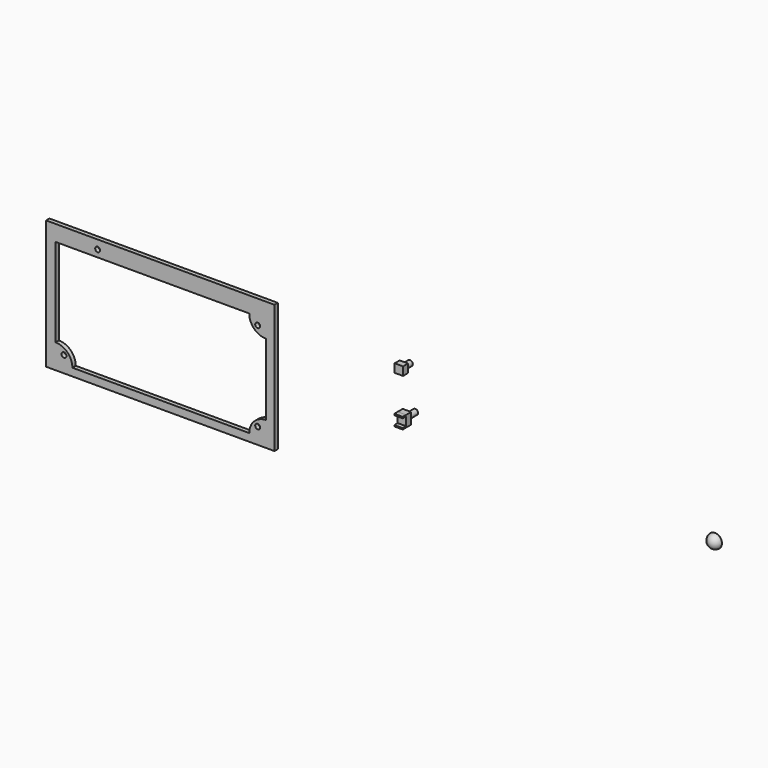
from build123d import *

# Parameters (mm, degrees)
F0_W      = 162.6942493021
F0_H      = 91.7676277459
F0_R      = 1.75
F1_DEPTH  = 3
F2_W      = 6
F2_H      = 6
F3_DEPTH  = 4.5
F4_R      = 1.95
F5_DEPTH  = 5.5
F6_W      = 6
F6_H      = 1
F7_DEPTH  = 3
F6_H_2    = 0.9
F8_W      = 6
F8_H      = 8
F9_DEPTH  = 4.5
F10_R     = 1.95
F11_DEPTH = 7.5


# Not quite as in the source:
# - a fillet or chamfer that OpenCascade refuses, or shapes differently, is made with other operations: its cross-section is extruded or revolved along the edge and cut away or added


with BuildPart() as f1:
    # F0 (on Front) → F1 (new body)
    with BuildSketch(Plane.XZ):
        with Locations((-36.5303959697, 18.2162802666)):
            Rectangle(F0_W, F0_H)
        with Locations((-105.142032113, -16.1853220011)):
            Circle(F0_R, mode=Mode.SUBTRACT)
        with Locations((32.857967887, -16.1853220011)):
            Circle(F0_R, mode=Mode.SUBTRACT)
        with BuildLine():
            Line((-111.142032113, -10.1853220011), (-111.142032113, 52.8146779989))
            Line((-111.142032113, 52.8146779989), (26.857967887, 52.8146779989))
            ThreePointArc((26.857967887, 52.8146779989), (30.3726865127, 44.3293966246), (38.857967887, 40.8146779989))
            Line((38.857967887, 40.8146779989), (38.857967887, -10.1853220011))
            ThreePointArc((38.857967887, -10.1853220011), (30.3726865127, -13.7000406269), (26.857967887, -22.1853220011))
            Line((26.857967887, -22.1853220011), (-99.142032113, -22.1853220011))
            ThreePointArc((-99.142032113, -22.1853220011), (-102.6567507388, -13.7000406269), (-111.142032113, -10.1853220011))
        make_face(mode=Mode.SUBTRACT)
        with Locations((-81.142032113, 57.8146779989)):
            Circle(F0_R, mode=Mode.SUBTRACT)
        with Locations((32.857967887, 47.3146779989)):
            Circle(F0_R, mode=Mode.SUBTRACT)
    extrude(amount=F1_DEPTH)


with BuildPart() as f3:
    # F2 (on Front) → F3 (new body)
    with BuildSketch(Plane.XZ):
        with Locations((134.6271275282, 53.2519980073)):
            Rectangle(F2_W, F2_H)
    extrude(amount=F3_DEPTH)

    # F4 (on face) → F5 (join)
    with BuildSketch(Plane(origin=(0, 0, 0), x_dir=(-1, 0, 0), z_dir=(0, 1, 0))):
        with Locations((-134.6271275282, 53.2519980073)):
            Circle(F4_R)
    extrude(amount=F5_DEPTH)


with BuildPart() as f7:
    # F6 (on Front) → F7 (new body)
    with BuildSketch(Plane.XZ):
        with Locations((133.2053928375, 23.0518818647)):
            Rectangle(F6_W, F6_H)
    extrude(amount=F7_DEPTH)


with BuildPart() as f7b:
    # F6 (on Front) → F7, piece 2 (new body)
    with BuildSketch(Plane.XZ):
        with Locations((133.2053928375, 16.0018818647)):
            Rectangle(F6_W, F6_H_2)
    extrude(amount=F7_DEPTH)


with BuildPart() as f9:
    # F8 (on face) → F9 (new body)
    with BuildSketch(Plane(origin=(0, 0, 0), x_dir=(-1, 0, 0), z_dir=(0, 1, 0))):
        with Locations((-133.2053928375, 19.5518818647)):
            Rectangle(F8_W, F8_H)
    extrude(amount=F9_DEPTH)

    # F10 (on face) → F11 (join)
    with BuildSketch(Plane(origin=(0, 4.5, 0), x_dir=(-1, 0, 0), z_dir=(0, 1, 0))):
        with Locations((-133.2053928375, 19.5518818647)):
            Circle(F10_R)
    extrude(amount=F11_DEPTH)


with BuildPart() as f14:
    # F13 (on face) → F14 (revolve)
    with BuildSketch(Plane.XY.offset(25)):
        with BuildLine():
            Line((366.844489096, -14.9696936347), (366.844489096, -17.9696936347))
            ThreePointArc((366.844489096, -17.9696936347), (370.3800230019, -16.5052275406), (371.844489096, -12.9696936347))
            Line((371.844489096, -12.9696936347), (368.844489096, -12.9696936347))
            Line((368.844489096, -12.9696936347), (368.844489096, -14.9696936347))
            Line((368.844489096, -14.9696936347), (366.844489096, -14.9696936347))
        make_face()
    revolve(axis=Axis((366.844489096, -20.7170091908, 25), (0, -1, 0)))

    # F15: chamfer of 0.3 on 2 edges, made by hand

    # F15_s1 → F15_t2 (revolve, cut)
    with BuildSketch(Plane.XY.offset(25)):
        Polygon((369.144489096, -12.9696936347), (368.844489096, -13.2696936347), (368.844489096, -12.9696936347), align=None)
    revolve(axis=Axis((366.844489096, -12.9696936347, 25), (0, -1, 0)), mode=Mode.SUBTRACT)

    # F15_s3 → F15_t4 (revolve, cut)
    with BuildSketch(Plane.XY.offset(25)):
        with BuildLine():
            Line((371.5349048558, -12.9696936347), (371.8342930958, -13.2888425708))
            ThreePointArc((371.8342930958, -13.2888425708), (371.8418022214, -13.133588499), (371.844489096, -12.9696936347))
            Line((371.844489096, -12.9696936347), (371.5349048558, -12.9696936347))
        make_face()
    revolve(axis=Axis((366.844489096, -12.9696936347, 25), (0, -1, 0)), mode=Mode.SUBTRACT)


solid = Compound([f1.part, f3.part, f7.part, f7b.part, f9.part, f14.part])
